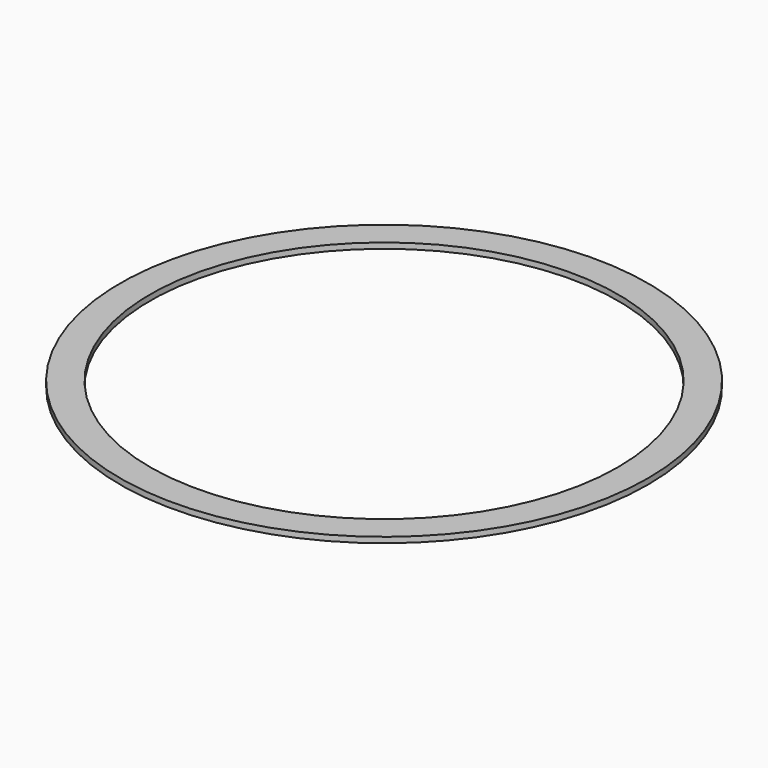
from build123d import *

# Parameters (mm, degrees)
F0_R     = 223.52508
F0_R_2   = 198.12508
F1_DEPTH = 4.7625


# Not quite as in the source:
# - a length typed as a fraction of an inch, garbled in the dataset ("3 / 203.2 mm" for 3/8 in), is restored


with BuildPart() as f1:
    # F0 (on Top) → F1 (new body)
    with BuildSketch(Plane.XY):
        Circle(F0_R)
        Circle(F0_R_2, mode=Mode.SUBTRACT)
    extrude(amount=F1_DEPTH)


solid = f1.part
